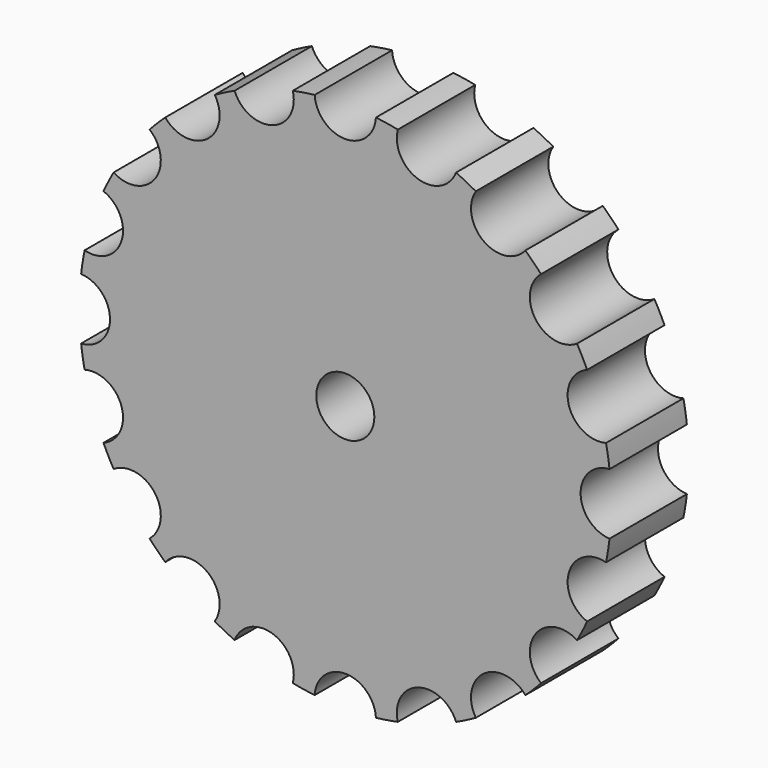
from build123d import *

# Parameters (mm, degrees)
F0_R            = 27.5
F0_R_2          = 3
F1_DEPTH        = 10
F2_R            = 3.17
F3_DEPTH        = 10.001
F3_COPIES_COUNT = 20


# Not quite as in the source:
# - a pattern or mirror of a feature is missing from the dataset's text; its kind, count and spacing are read off the source's solid


with BuildPart() as f1:
    # F0 (on Front) → F1 (new body)
    with BuildSketch(Plane.XZ):
        Circle(F0_R)
        Circle(F0_R_2, mode=Mode.SUBTRACT)
    extrude(amount=F1_DEPTH)

    # F2 (on face) → F3 (cut, through all)
    with BuildSketch(Plane.XZ.offset(10)):
        with Locations((0, 27.5)):
            Circle(F2_R)
    f3 = extrude(amount=-F3_DEPTH, mode=Mode.SUBTRACT)

    # F3_copies: F3 ×20 about axis
    f3_copies_axis = Axis((0, 0, 0), (0, 1, 0))
    for i in range(1, F3_COPIES_COUNT):
        add(f3.rotate(f3_copies_axis, i * 360 / F3_COPIES_COUNT), mode=Mode.SUBTRACT)


solid = f1.part
